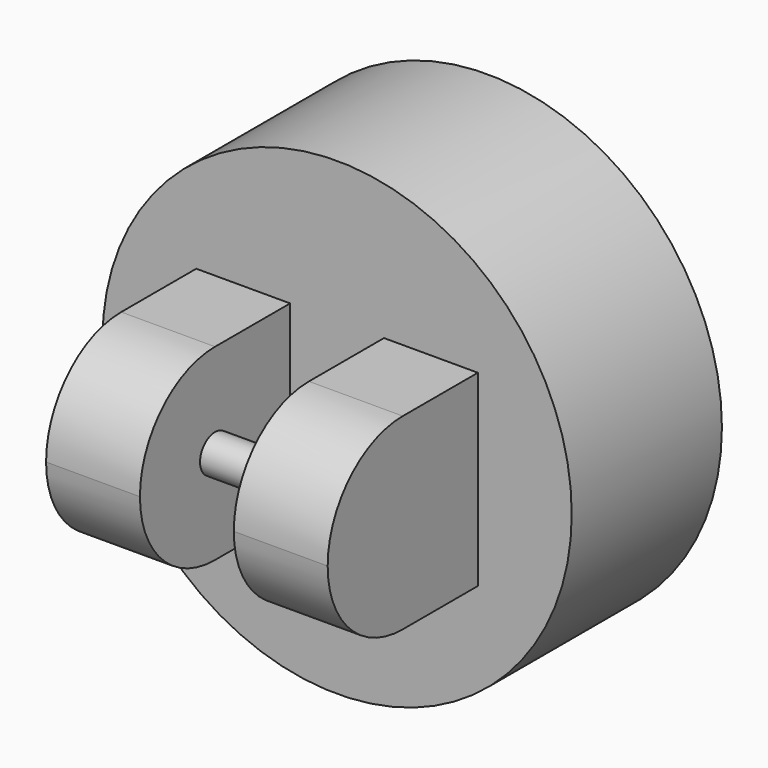
from build123d import *

# Parameters (mm, degrees)
F0_R     = 15.875
F1_DEPTH = 12.7
F2_W     = 6.35
F2_H     = 12.7
F3_DEPTH = 12.7
F4_R     = 6.34999
F5_R     = 1.27
F6_DEPTH = 19.05


# Not quite as in the source:
# - a fillet or chamfer is up to 0.001 mm smaller than in the source, because OpenCascade refuses the exact size


with BuildPart() as f1:
    # F0 (on Front) → F1 (new body)
    with BuildSketch(Plane.XZ):
        Circle(F0_R)
    extrude(amount=-F1_DEPTH)

    # F2 (on face) → F3 (join)
    with BuildSketch(Plane.XZ):
        with Locations((-6.35, 0)):
            Rectangle(F2_W, F2_H)
        with Locations((6.35, 0)):
            Rectangle(F2_W, F2_H)
    extrude(amount=F3_DEPTH)

    # F4 (radius 6.35 in the source; OpenCascade refuses exactly that, so slightly less here)
    f4_edges = [f1.edges().sort_by_distance(p)[0] for p in [
        (-6.35, -12.7, 6.35),
        (6.35, -12.7, 6.35),
        (-6.35, -12.7, -6.35),
        (6.35, -12.7, -6.35),
    ]]
    fillet(f4_edges, radius=F4_R)

    # F5 (on face) → F6 (join)
    with BuildSketch(Plane.YZ.offset(9.525)):
        with Locations((-6.35, 0)):
            Circle(F5_R)
    extrude(amount=-F6_DEPTH)


solid = f1.part
